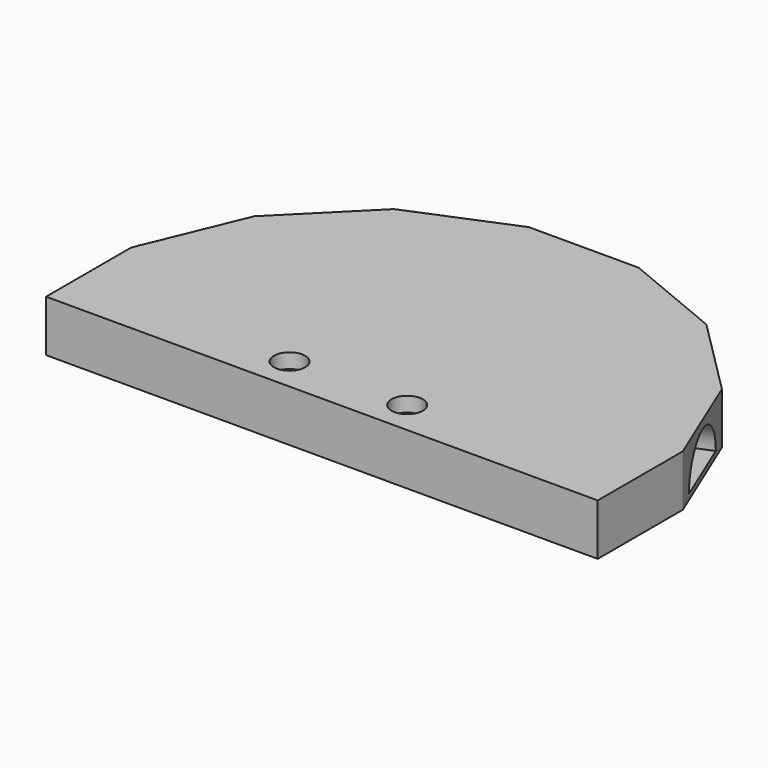
from build123d import *

# Parameters (mm, degrees)
F0_W      = 150
F0_H      = 10
F0_R      = 2.25
F1_DEPTH  = 14
F5_DEPTH  = 15
F6_DEPTH  = 15
F7_DEPTH  = 15
F8_R      = 4.25
F9_DEPTH  = 4
F10_W     = 150
F10_H     = 14
F11_DEPTH = 4
F12_R     = 4.25
F13_DEPTH = 3
F14_R     = 1
F17_DEPTH = 15
F18_DEPTH = 15
F21_DEPTH = 15
F22_DEPTH = 15


with BuildPart() as f1:
    # F0 (on Top) → F1 (new body)
    with BuildSketch(Plane.XY):
        Polygon((0, 14.9184275535), (0, 0), (150, 0), (150, 14.9184275535), (138.5819298767, 42.4840873013), (117.4840873013, 63.5819298767), (89.9184275535, 75), (60.0815724465, 75), (32.5159126987, 63.5819298767), (11.4180701233, 42.4840873013), align=None)
        with Locations((75, -5)):
            Rectangle(F0_W, F0_H)
        with Locations((59, -5)):
            Circle(F0_R, mode=Mode.SUBTRACT)
        with Locations((91, -5)):
            Circle(F0_R, mode=Mode.SUBTRACT)
    extrude(amount=F1_DEPTH)

    # F4 (on face) → F5 (cut)
    with BuildSketch(Plane(origin=(90.533008589, 90.533008589, 0), x_dir=(-0.7071067812, 0.7071067812, 0), z_dir=(0.7071067812, 0.7071067812, 0))):
        with BuildLine():
            ThreePointArc((-42.783008589, 1.5), (-53.033008589, 11.75), (-63.283008589, 1.5))
            Line((-63.283008589, 1.5), (-42.783008589, 1.5))
        make_face()
    extrude(amount=-F5_DEPTH, mode=Mode.SUBTRACT)

    # F2 (on face) → F6 (cut)
    with BuildSketch(Plane(origin=(0, 75, 0), x_dir=(-1, 0, 0), z_dir=(0, 1, 0))):
        with BuildLine():
            ThreePointArc((-64.75, 1.5), (-75, 11.75), (-85.25, 1.5))
            Line((-85.25, 1.5), (-64.75, 1.5))
        make_face()
    extrude(amount=-F6_DEPTH, mode=Mode.SUBTRACT)

    # F3 (on face) → F7 (cut)
    with BuildSketch(Plane(origin=(-15.533008589, 15.533008589, 0), x_dir=(-0.7071067812, -0.7071067812, 0), z_dir=(-0.7071067812, 0.7071067812, 0))):
        with BuildLine():
            ThreePointArc((-42.783008589, 1.5), (-53.033008589, 11.75), (-63.283008589, 1.5))
            Line((-63.283008589, 1.5), (-42.783008589, 1.5))
        make_face()
    extrude(amount=-F7_DEPTH, mode=Mode.SUBTRACT)

    # F8 (on face) → F9 (cut)
    with BuildSketch(Plane.XY.offset(14)):
        with Locations((59, -5)):
            Circle(F8_R)
        with Locations((91, -5)):
            Circle(F8_R)
    extrude(amount=-F9_DEPTH, mode=Mode.SUBTRACT)

    # F10 (on face) → F11 (join)
    with BuildSketch(Plane.XZ.offset(10)):
        with Locations((75, 7)):
            Rectangle(F10_W, F10_H)
    extrude(amount=F11_DEPTH)

    # F12 (on face) → F13 (cut)
    with BuildSketch(Plane(origin=(0, 0, 0), x_dir=(1, 0, 0), z_dir=(0, 0, -1))):
        with Locations((75, -37)):
            Circle(F12_R)
    extrude(amount=-F13_DEPTH, mode=Mode.SUBTRACT)

    # F14
    f14_edges = [f1.edges().sort_by_distance(p)[0] for p in [
        (70.75, 37, 0),
        (70.75, 37, 3),
    ]]
    fillet(f14_edges, radius=F14_R)

    # F16 (on face) → F17 (cut)
    with BuildSketch(Plane(origin=(133.3074692328, 55.2177617219, 0), x_dir=(-0.3826834324, 0.9238795325, 0), z_dir=(0.9238795325, 0.3826834324, 0))):
        with BuildLine():
            ThreePointArc((-18.4512574274, 1.5), (-28.7012574274, 11.75), (-38.9512574274, 1.5))
            Line((-38.9512574274, 1.5), (-18.4512574274, 1.5))
        make_face()
    extrude(amount=-F17_DEPTH, mode=Mode.SUBTRACT)

    # F15 (on face) → F18 (cut)
    with BuildSketch(Plane(origin=(-5.2744606439, 2.1847531329, 0), x_dir=(-0.3826834324, -0.9238795325, 0), z_dir=(-0.9238795325, 0.3826834324, 0))):
        with BuildLine():
            ThreePointArc((-18.4512574274, 1.5), (-28.7012574274, 11.75), (-38.9512574274, 1.5))
            Line((-38.9512574274, 1.5), (-18.4512574274, 1.5))
        make_face()
    extrude(amount=-F18_DEPTH, mode=Mode.SUBTRACT)

    # F20 (on face) → F21 (cut)
    with BuildSketch(Plane(origin=(-17.7177617219, 42.7744606439, 0), x_dir=(-0.9238795325, -0.3826834324, 0), z_dir=(-0.3826834324, 0.9238795325, 0))):
        with BuildLine():
            ThreePointArc((-59.0409649383, 1.5), (-69.2909649383, 11.75), (-79.5409649383, 1.5))
            Line((-79.5409649383, 1.5), (-59.0409649383, 1.5))
        make_face()
    extrude(amount=-F21_DEPTH, mode=Mode.SUBTRACT)

    # F19 (on face) → F22 (cut)
    with BuildSketch(Plane(origin=(39.6847531329, 95.8074692328, 0), x_dir=(-0.9238795325, 0.3826834324, 0), z_dir=(0.3826834324, 0.9238795325, 0))):
        with BuildLine():
            ThreePointArc((-59.0409649383, 1.5), (-69.2909649383, 11.75), (-79.5409649383, 1.5))
            Line((-79.5409649383, 1.5), (-59.0409649383, 1.5))
        make_face()
    extrude(amount=-F22_DEPTH, mode=Mode.SUBTRACT)


solid = f1.part
